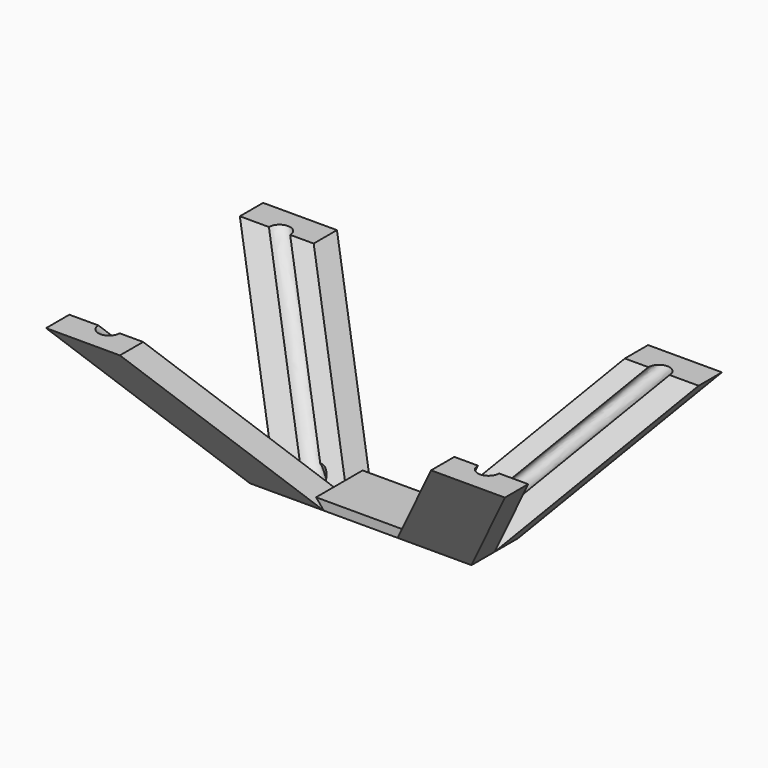
from build123d import *

# Parameters (mm, degrees)
F0_W           = 10
F0_H           = 7.875
F1_DEPTH       = 2.5
F11_DEPTH      = 25
F13_DEPTH      = 7.875
F13_DEPTH_BACK = 7.875


with BuildPart() as f1:
    # F0 (on Top) → F1 (new body)
    with BuildSketch(Plane.XY):
        with Locations((-5, 3.9375)):
            Rectangle(F0_W, F0_H)
        with Locations((5, 3.9375)):
            Rectangle(F0_W, F0_H)
        with Locations((5, -3.9375)):
            Rectangle(F0_W, F0_H)
        with Locations((-5, -3.9375)):
            Rectangle(F0_W, F0_H)
    extrude(amount=F1_DEPTH)

    # F8: sweep along a path in F4
    with BuildLine(Plane(origin=(-5.8682408883, 0, -4.9240387651), x_dir=(0, 1, 0), z_dir=(0.7660444431, 0, 0.6427876097))) as f8_path:
        Line((-28.8675134595, 56.6363319121), (0, 6.6363319121))
    # F0 (on Top) → F8 (sweep)
    with BuildSketch(Plane.XY):
        with BuildLine():
            Line((-10, 0), (-16.375, 0))
            ThreePointArc((-16.375, 0), (-19.25, -2.875), (-22.125, 0))
            Line((-22.125, 0), (-30, 0))
            Line((-30, 0), (-30, -7.875))
            Line((-30, -7.875), (-10, -7.875))
            Line((-10, -7.875), (-10, 0))
        make_face()
    sweep(path=f8_path.line)

    # F10: sweep along a path in F7
    with BuildLine(Plane(origin=(5.8682408883, 0, -4.9240387651), x_dir=(0, 1, 0), z_dir=(0.7660444431, 0, -0.6427876097))) as f10_path:
        Line((28.8675134595, 56.5418889989), (0, 6.5418889989))
    # F0 (on Top) → F10 (sweep)
    with BuildSketch(Plane.XY):
        with BuildLine():
            Line((10, 7.875), (10, 0))
            Line((10, 0), (16.375, 0))
            ThreePointArc((16.375, 0), (19.25, 2.875), (22.125, 0))
            Line((22.125, 0), (30, 0))
            Line((30, 0), (30, 7.875))
            Line((30, 7.875), (10, 7.875))
        make_face()
    sweep(path=f10_path.line)


with BuildPart() as f5:
    # F5: sweep along a path in F4
    with BuildLine(Plane(origin=(-5.8682408883, 0, -4.9240387651), x_dir=(0, 1, 0), z_dir=(0.7660444431, 0, 0.6427876097))) as f5_path:
        Line((28.8675134595, 56.6363319121), (0, 6.6363319121))
    # F0 (on Top) → F5 (sweep)
    with BuildSketch(Plane.XY):
        with BuildLine():
            ThreePointArc((-22.125, 0), (-19.25, 2.875), (-16.375, 0))
            Line((-16.375, 0), (-10, 0))
            Line((-10, 0), (-10, 7.875))
            Line((-10, 7.875), (-30, 7.875))
            Line((-30, 7.875), (-30, 0))
            Line((-30, 0), (-22.125, 0))
        make_face()
    sweep(path=f5_path.line)


with BuildPart() as f9:
    # F9: sweep along a path in F7
    with BuildLine(Plane(origin=(5.8682408883, 0, -4.9240387651), x_dir=(0, 1, 0), z_dir=(0.7660444431, 0, -0.6427876097))) as f9_path:
        Line((-28.8675134595, 56.5418889989), (0, 6.5418889989))
    # F0 (on Top) → F9 (sweep)
    with BuildSketch(Plane.XY):
        with BuildLine():
            Line((16.375, 0), (10, 0))
            Line((10, 0), (10, -7.875))
            Line((10, -7.875), (30, -7.875))
            Line((30, -7.875), (30, 0))
            Line((30, 0), (22.125, 0))
            ThreePointArc((22.125, 0), (19.25, -2.875), (16.375, 0))
        make_face()
    sweep(path=f9_path.line)


with BuildPart() as f11_tool:
    # F0 (on Top) → F11 (new body)
    with BuildSketch(Plane.XY):
        with BuildLine():
            Line((19.25, 0), (16.375, 0))
            ThreePointArc((16.375, 0), (19.25, -2.875), (22.125, 0))
            Line((22.125, 0), (19.25, 0))
        make_face()
        with BuildLine():
            ThreePointArc((22.125, 0), (19.25, 2.875), (16.375, 0))
            Line((16.375, 0), (19.25, 0))
            Line((19.25, 0), (22.125, 0))
        make_face()
        with BuildLine():
            Line((-22.125, 0), (-19.25, 0))
            Line((-19.25, 0), (-16.375, 0))
            ThreePointArc((-16.375, 0), (-19.25, 2.875), (-22.125, 0))
        make_face()
        with BuildLine():
            Line((-16.375, 0), (-19.25, 0))
            Line((-19.25, 0), (-22.125, 0))
            ThreePointArc((-22.125, 0), (-19.25, -2.875), (-16.375, 0))
        make_face()
    extrude(amount=F11_DEPTH)


with BuildPart() as f1_1:
    add(f1.part)

    # F11: cut by f11_tool
    add(f11_tool.part, mode=Mode.SUBTRACT)

    # F12 (on Front) → F13 (join, two sides)
    with BuildSketch(Plane.XZ) as f13_sk:
        Polygon((10, 2.5), (10, 0), (12.0977490779, 2.5), align=None)
        Polygon((-12.0977490779, 2.5), (-10, 0), (-10, 2.5), align=None)
    extrude(amount=F13_DEPTH)
    extrude(f13_sk.sketch, amount=-F13_DEPTH_BACK)


with BuildPart() as f5_1:
    add(f5.part)

    # F11: cut by f11_tool
    add(f11_tool.part, mode=Mode.SUBTRACT)


with BuildPart() as f9_1:
    add(f9.part)

    # F11: cut by f11_tool
    add(f11_tool.part, mode=Mode.SUBTRACT)


solid = Compound([f1_1.part, f5_1.part, f9_1.part])
